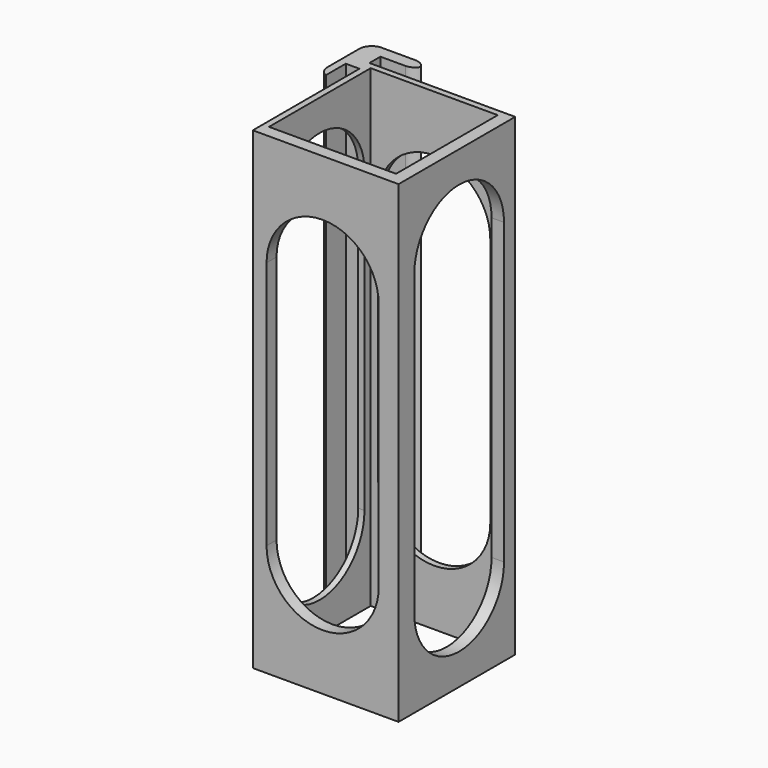
from build123d import *

# Parameters (mm, degrees)
F0_W        = 5.5
F0_H        = 5
F0_W_2      = 51
F0_H_2      = 51
F1_DEPTH    = 190
F2_T1_DEPTH = 215
F2_T3_DEPTH = 212.9128784748
F4_DEPTH    = 60
F6_DEPTH    = 60


# Not quite as in the source:
# - a fillet or chamfer that OpenCascade refuses, or shapes differently, is made with other operations: its cross-section is extruded or revolved along the edge and cut away or added


with BuildPart() as f1:
    # F0 (on Top) → F1 (new body)
    with BuildSketch(Plane.XY):
        Polygon((-33.5212003861, 28.1146157656), (-28.0212003861, 28.1146157656), (-28.0212003861, 33.6146157656), (-28.0212003861, 38.6146157656), (-36.5212003861, 38.6146157656), (-36.5212003861, 28.1146157656), align=None)
        Polygon((-28.0212003861, 38.6146157656), (-28.0212003861, 33.6146157656), (-23.0212003861, 33.6146157656), (-13.0212003861, 33.6146157656), (-13.0212003861, 38.6146157656), align=None)
        with Locations((-30.7712003861, 25.6146157656)):
            Rectangle(F0_W, F0_H)
        Polygon((-33.5212003861, 23.1146157656), (-33.5212003861, 28.1146157656), (-36.5212003861, 28.1146157656), (-36.5212003861, 13.1146157656), (-33.5212003861, 13.1146157656), align=None)
        Polygon((-23.0212003861, 28.1146157656), (-28.0212003861, 28.1146157656), (-28.0212003861, 23.1146157656), (-28.0212003861, -30.3853842344), (30.4787996139, -30.3853842344), (30.4787996139, 28.1146157656), align=None)
        with Locations((-0.0212003861, 0.1146157656)):
            Rectangle(F0_W_2, F0_H_2, mode=Mode.SUBTRACT)
    extrude(amount=F1_DEPTH)

    # F2: fillet of radius 5 on 4 edges, made by hand

    # F2_s2 → F2_t1 (cut)
    with BuildSketch(Plane.XY.offset(-12.5)):
        with BuildLine():
            ThreePointArc((-31.5212003861, 38.6146157656), (-35.056734292, 37.1501496716), (-36.5212003861, 33.6146157656))
            Line((-36.5212003861, 33.6146157656), (-36.5212003861, 38.6146157656))
            Line((-36.5212003861, 38.6146157656), (-31.5212003861, 38.6146157656))
        make_face()
        with BuildLine():
            ThreePointArc((-13.0212003861, 33.6146157656), (-14.4856664802, 37.1501496716), (-18.0212003861, 38.6146157656))
            Line((-18.0212003861, 38.6146157656), (-13.0212003861, 38.6146157656))
            Line((-13.0212003861, 38.6146157656), (-13.0212003861, 33.6146157656))
        make_face()
        with BuildLine():
            ThreePointArc((-18.0212003861, 33.6146157656), (-14.4856664802, 35.0790818597), (-13.0212003861, 38.6146157656))
            Line((-13.0212003861, 38.6146157656), (-13.0212003861, 33.6146157656))
            Line((-13.0212003861, 33.6146157656), (-18.0212003861, 33.6146157656))
        make_face()
    extrude(amount=F2_T1_DEPTH, mode=Mode.SUBTRACT)

    # F2_s4 → F2_t3 (cut)
    with BuildSketch(Plane.XY.offset(-11.4564392374)):
        with BuildLine():
            ThreePointArc((-36.5212003861, 17.6971914606), (-35.7045005188, 14.9585786731), (-33.5212003861, 13.1146157656))
            Line((-33.5212003861, 13.1146157656), (-36.5212003861, 13.1146157656))
            Line((-36.5212003861, 13.1146157656), (-36.5212003861, 17.6971914606))
        make_face()
    extrude(amount=F2_T3_DEPTH, mode=Mode.SUBTRACT)

    # F3 (on face) → F4 (cut)
    with BuildSketch(Plane.YZ.offset(30.4787996139)):
        with BuildLine():
            Line((-22.5, 155), (22.5, 155))
            ThreePointArc((22.5, 155), (0, 177.5), (-22.5, 155))
        make_face()
        with BuildLine():
            ThreePointArc((-22.5, 155), (0, 132.5), (22.5, 155))
            Line((22.5, 155), (-22.5, 155))
        make_face()
        with BuildLine():
            ThreePointArc((-22.5, 35), (0, 57.5), (22.5, 35))
            Line((22.5, 35), (22.5, 155))
            ThreePointArc((22.5, 155), (0, 132.5), (-22.5, 155))
            Line((-22.5, 155), (-22.5, 35))
        make_face()
        with BuildLine():
            Line((-22.5, 35), (22.5, 35))
            ThreePointArc((22.5, 35), (0, 57.5), (-22.5, 35))
        make_face()
        with BuildLine():
            ThreePointArc((-22.5, 35), (0, 12.5), (22.5, 35))
            Line((22.5, 35), (-22.5, 35))
        make_face()
    extrude(amount=-F4_DEPTH, mode=Mode.SUBTRACT)

    # F5 (on face) → F6 (cut)
    with BuildSketch(Plane.XZ.offset(30.3853842344)):
        with BuildLine():
            Line((-22.5, 145), (22.5, 145))
            ThreePointArc((22.5, 145), (0, 167.5), (-22.5, 145))
        make_face()
        with BuildLine():
            ThreePointArc((-22.5, 145), (0, 122.5), (22.5, 145))
            Line((22.5, 145), (-22.5, 145))
        make_face()
        with BuildLine():
            Line((22.5, 45), (22.5, 145))
            ThreePointArc((22.5, 145), (0, 122.5), (-22.5, 145))
            Line((-22.5, 145), (-22.5, 45))
            ThreePointArc((-22.5, 45), (0, 67.5), (22.5, 45))
        make_face()
        with BuildLine():
            Line((-22.5, 45), (22.5, 45))
            ThreePointArc((22.5, 45), (0, 67.5), (-22.5, 45))
        make_face()
        with BuildLine():
            ThreePointArc((-22.5, 45), (0, 22.5), (22.5, 45))
            Line((22.5, 45), (-22.5, 45))
        make_face()
    extrude(amount=-F6_DEPTH, mode=Mode.SUBTRACT)


solid = f1.part
